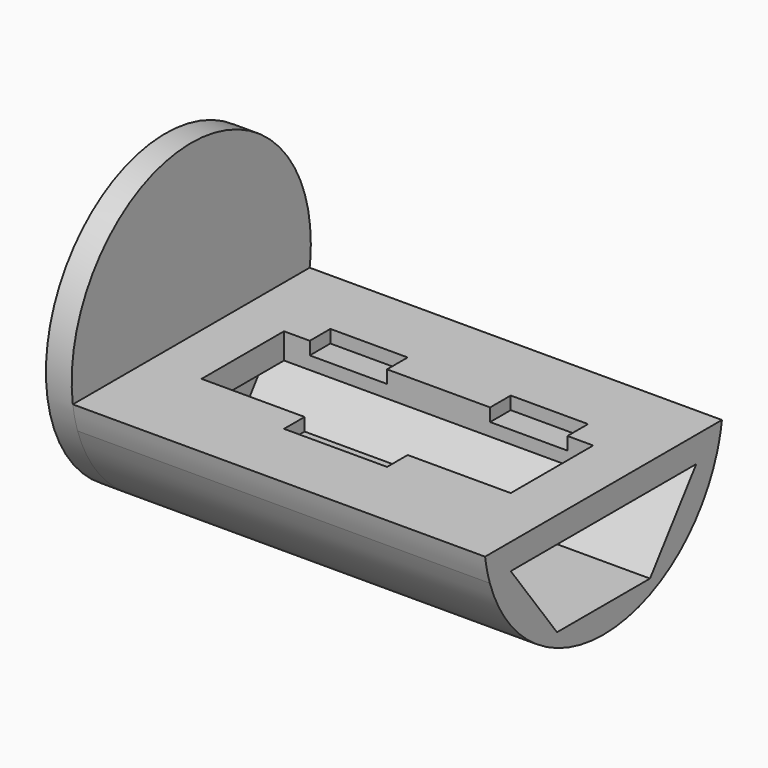
from build123d import *

# Parameters (mm, degrees)
F2_DEPTH = 101.6
F0_R     = 36.83
F3_DEPTH = 6.35
F5_DEPTH = 6.35
F6_DEPTH = 3.175


# Not quite as in the source:
# - a feature names something its author has since deleted; it is built from what else it names


with BuildPart() as f2:
    # F1 (on face) → F2 (new body)
    with BuildSketch(Plane.YZ):
        Polygon((-28.5745194683, -8.2572300072), (-28.5730573626, -11.4344600145), (-18.8812190642, -11.43), (-6.2808282673, -11.43), (-6.2808282673, -8.2563601018), align=None)
        Polygon((0, -8.2561150224), (0, -11.43), (12.7450705782, -11.43), (28.5754804883, -11.43), (28.5754804883, -8.255), align=None)
        with BuildLine():
            Line((-14.324102157, -30.48), (-20.674102157, -30.48))
            ThreePointArc((-20.674102157, -30.48), (-10.8136603424, -35.2067273401), (0, -36.83))
            Line((0, -36.83), (0, -30.48))
            Line((0, -30.48), (-14.324102157, -30.48))
        make_face()
        with BuildLine():
            Line((0, -30.48), (0, -36.83))
            ThreePointArc((0, -36.83), (10.8136603424, -35.2067273401), (20.674102157, -30.48))
            Line((20.674102157, -30.48), (14.324102157, -30.48))
            Line((14.324102157, -30.48), (0, -30.48))
        make_face()
        Polygon((-6.2808282673, -11.43), (0, -11.43), (0, -8.2561150224), (-6.2808282673, -8.2563601018), align=None)
        Polygon((-6.2808282673, -8.2563601018), (0, -8.2561150224), (0, -5.08), (-6.2808282673, -5.08), align=None)
        with BuildLine():
            ThreePointArc((-36.4779728055, -5.08), (-35.8845812082, -8.2913045723), (-35.0090600232, -11.4374217503))
            Line((-35.0090600232, -11.4374217503), (-28.5730573626, -11.4344600145))
            Line((-28.5730573626, -11.4344600145), (-28.5745194683, -8.2572300072))
            Line((-28.5745194683, -8.2572300072), (-28.5759815739, -5.08))
            Line((-28.5759815739, -5.08), (-36.4779728055, -5.08))
        make_face()
        Polygon((-28.5759815739, -5.08), (-28.5745194683, -8.2572300072), (-6.2808282673, -8.2563601018), (-6.2808282673, -5.08), align=None)
        Polygon((0, -5.08), (0, -8.2561150224), (28.5754804883, -8.255), (28.5754804883, -5.08), align=None)
        with BuildLine():
            Line((28.5754804883, -11.43), (35.0114838303, -11.43))
            ThreePointArc((35.0114838303, -11.43), (35.8854598343, -8.2875009791), (36.4779728055, -5.08))
            Line((36.4779728055, -5.08), (28.5754804883, -5.08))
            Line((28.5754804883, -5.08), (28.5754804883, -8.255))
            Line((28.5754804883, -8.255), (28.5754804883, -11.43))
        make_face()
        with BuildLine():
            Line((14.324102157, -30.48), (20.674102157, -30.48))
            ThreePointArc((20.674102157, -30.48), (29.4269731146, -22.1472832038), (35.0114838303, -11.43))
            Line((35.0114838303, -11.43), (28.5754804883, -11.43))
            Line((28.5754804883, -11.43), (14.324102157, -30.48))
        make_face()
        with BuildLine():
            ThreePointArc((-35.0090600232, -11.4374217503), (-29.4246254725, -22.150402159), (-20.674102157, -30.48))
            Line((-20.674102157, -30.48), (-14.324102157, -30.48))
            Line((-14.324102157, -30.48), (-28.5730573626, -11.4344600145))
            Line((-28.5730573626, -11.4344600145), (-35.0090600232, -11.4374217503))
        make_face()
    extrude(amount=F2_DEPTH)

    # F0 (on Right) → F3 (join)
    with BuildSketch(Plane.YZ):
        Circle(F0_R)
    extrude(amount=-F3_DEPTH)

    # F4 (on face) → F5 (cut)
    with BuildSketch(Plane.XY.offset(-5.08)):
        Polygon((19.05, 12.7), (12.7, 12.7), (12.7, 0), (12.7, -12.7), (38.1, -12.7), (50.8, -12.7), (63.5, -12.7), (88.9, -12.7), (88.9, 0), (88.9, 12.7), (82.55, 12.7), (63.5, 12.7), (50.8, 12.7), (38.1, 12.7), align=None)
    extrude(amount=-F5_DEPTH, mode=Mode.SUBTRACT)

    # F4 (on face) → F6 (cut)
    with BuildSketch(Plane.XY.offset(-5.08)):
        Polygon((19.05, 15.875), (19.05, 12.7), (38.1, 12.7), (38.1, 15.875), (38.1, 19.05), (19.05, 19.05), align=None)
        Polygon((50.8, -12.7), (38.1, -12.7), (38.1, -15.875), (38.1, -19.05), (63.5, -19.05), (63.5, -15.875), (63.5, -12.7), align=None)
        Polygon((63.5, 15.875), (63.5, 12.7), (82.55, 12.7), (82.55, 15.875), (82.55, 19.05), (63.5, 19.05), align=None)
    extrude(amount=-F6_DEPTH, mode=Mode.SUBTRACT)


solid = f2.part
